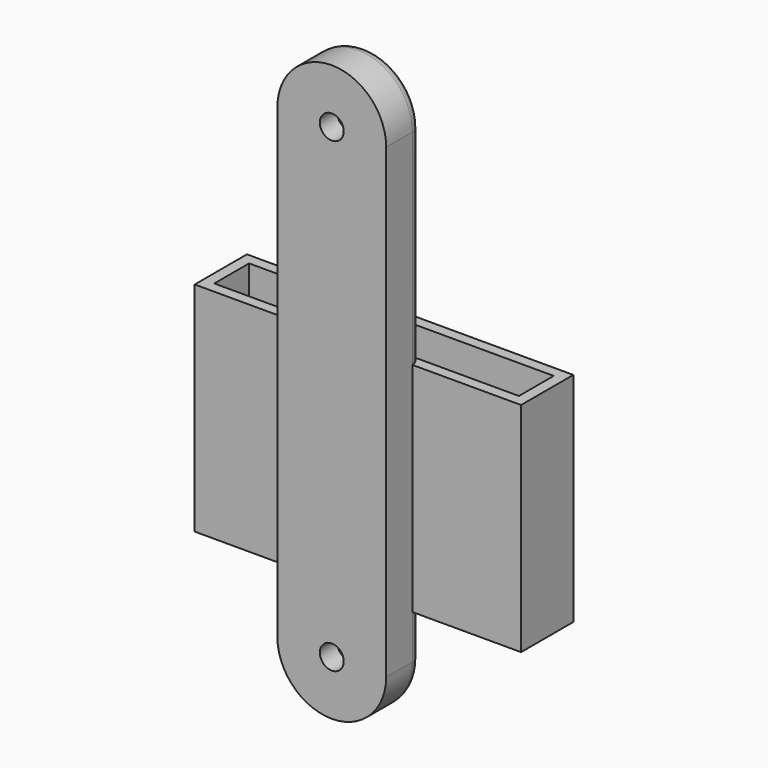
from build123d import *

# Parameters (mm, degrees)
F0_W           = 56
F0_H           = 8
F1_DEPTH       = 20
F2_START       = -14.9
F2_DEPTH       = 4.8
F4_DEPTH       = 8
F5_R           = 2
F7_D           = 4.4
F7_CBORE_D     = 8.25
F7_CBORE_DEPTH = 4


# Not quite as in the source:
# - a feature of the source that left no trace in its solid (it failed there, or was rolled back) is left out


with BuildPart() as f1:
    # F0 (on Top) → F1 (new body, symmetric)
    with BuildSketch(Plane.XY):
        Polygon((-26.7077493668, 10), (-46.7077493668, 10), (-46.7077493668, -2), (13.2922506332, -2), (13.2922506332, 10), (-6.7077493668, 10), align=None)
        with Locations((-16.7077493668, 4)):
            Rectangle(F0_W, F0_H, mode=Mode.SUBTRACT)
    extrude(amount=F1_DEPTH, both=True)

    # F0 (on Top) → F2 (join)
    with BuildSketch(Plane.XY.offset(F2_START)):
        with Locations((-16.7077493668, 4)):
            Rectangle(F0_W, F0_H)
    extrude(amount=-F2_DEPTH)

    # F3 (on Front) → F4 (join)
    with BuildSketch(Plane.XZ):
        with BuildLine():
            Line((-26.7077493668, 57.6839694445), (-26.7077493668, -28.1024485154))
            ThreePointArc((-26.7077493668, -28.1024485154), (-16.7077493668, -38.1024485154), (-6.7077493668, -28.1024485154))
            Line((-6.7077493668, -28.1024485154), (-6.7077493668, 57.6839694445))
            ThreePointArc((-6.7077493668, 57.6839694445), (-16.7077493668, 67.6839694445), (-26.7077493668, 57.6839694445))
        make_face()
    extrude(amount=F4_DEPTH)

    # F5
    f5_edges = [f1.edges().sort_by_distance(p)[0] for p in [
        (-16.707749, 0, 67.683969),
        (-6.707749, 0, 38.841985),
        (-6.707749, 0, -24.051224),
        (-26.707749, 0, 38.841985),
        (-26.707749, 0, -24.051224),
    ]]
    fillet(f5_edges, radius=F5_R)

    # F7 (through all)
    with Locations(Plane(origin=(0, 0, 0), x_dir=(1, 0, 0), z_dir=(0, 1, 0))):
        with Locations((-16.7077493668, -57.6839694445), (-16.7077493668, 28.1024485154)):
            CounterBoreHole(F7_D / 2, F7_CBORE_D / 2, F7_CBORE_DEPTH)


solid = f1.part
